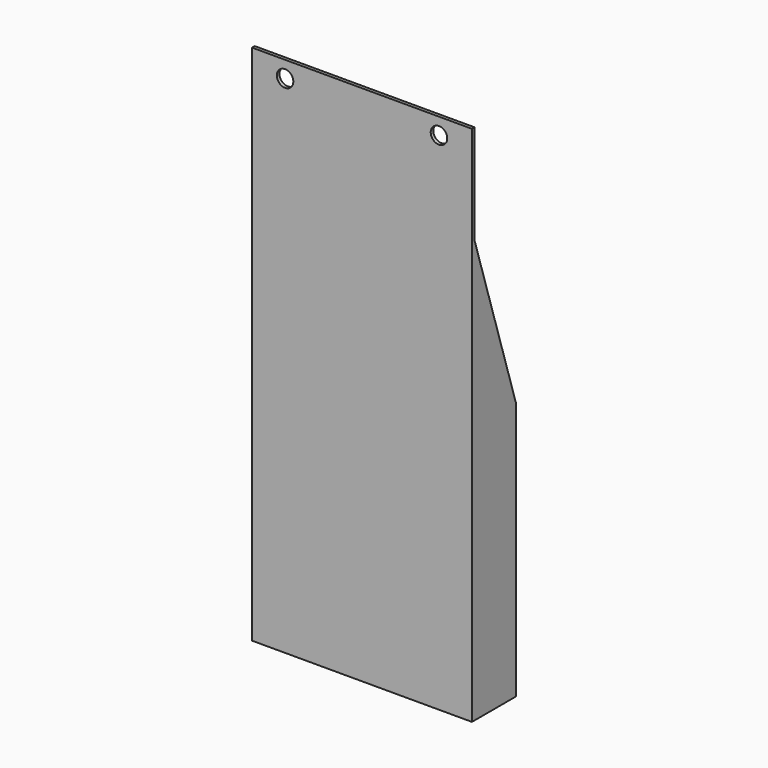
from build123d import *

# Parameters (mm, degrees)
F0_W          = 38
F0_H          = 46
F2_DEPTH      = 10
F0_R          = 1.5
F3_DEPTH      = 0.6
F4_R          = 2
F5_DEPTH      = 25
F5_DEPTH_BACK = 25


with BuildPart() as f2:
    # F0 (on Front) → F2 (new body)
    with BuildSketch(Plane.XZ):
        Polygon((19, -47.5), (20, -47.5), (20, 47.5), (19, 47.5), (19, 44.5), (19, 0.5), (-19, 0.5), (-19, 47.5), (-20, 47.5), (-20, -47.5), align=None)
        with Locations((0, -23.5)):
            Rectangle(F0_W, F0_H, mode=Mode.SUBTRACT)
    extrude(amount=-F2_DEPTH)

    # F0 (on Front) → F3 (join)
    with BuildSketch(Plane.XZ):
        Polygon((19, 44.5), (19, 47.5), (-19, 47.5), (-19, 0.5), (19, 0.5), align=None)
        with Locations((-14, 44.5)):
            Circle(F0_R, mode=Mode.SUBTRACT)
        with Locations((14, 44.5)):
            Circle(F0_R, mode=Mode.SUBTRACT)
        with Locations((0, -23.5)):
            Rectangle(F0_W, F0_H)
    extrude(amount=-F3_DEPTH)

    # F4
    f4_edges = [f2.edges().sort_by_distance(p)[0] for p in [
        (-19, 0.6, 24),
        (0, 0.6, 0.5),
        (19, 0.6, 24),
        (-19, 0.6, -23.5),
        (0, 0.6, -0.5),
        (19, 0.6, -23.5),
        (0, 0.6, -46.5),
    ]]
    fillet(f4_edges, radius=F4_R)

    # F1 (on Right) → F5 (cut, two sides)
    with BuildSketch(Plane.YZ) as f5_sk:
        Polygon((10, -0.4571680084), (10, 31.2587800152), (10, 64.4635409117), (1, 64.4635409117), (0.6, 64.4635409117), (0.6, 29.3558231338), (1, 28.0871852128), (9.8558554806, 0), align=None)
    extrude(amount=-F5_DEPTH, mode=Mode.SUBTRACT)
    extrude(f5_sk.sketch, amount=F5_DEPTH_BACK, mode=Mode.SUBTRACT)


solid = f2.part
